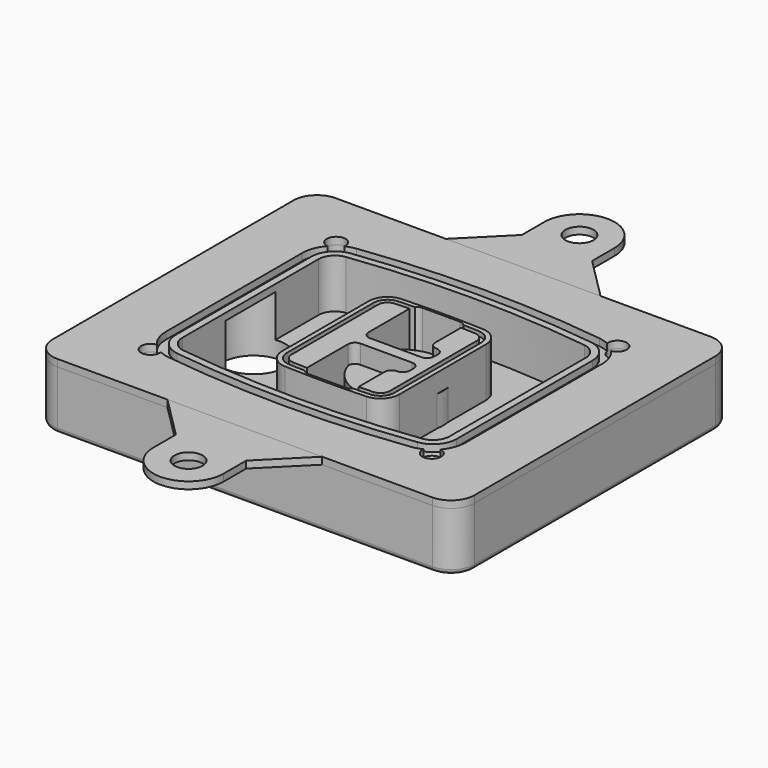
from build123d import *

# Parameters (mm, degrees)
F1_DEPTH  = 25
F2_DEPTH  = 3
F3_DEPTH  = 18
F5_DEPTH  = 21
F6_DEPTH  = 2
F8_DEPTH  = 20
F9_DEPTH  = 16
F10_DEPTH = 25
F7_R      = 6
F7_R_2    = 4
F11_DEPTH = 6
F13_DEPTH = 9
F15_R     = 2
F17_DEPTH = 3
F16_R     = 6


# Not quite as in the source:
# - a feature of the source that left no trace in its solid (it failed there, or was rolled back) is left out
# - a feature names something its author has since deleted; it is built from what else it names


with BuildPart() as f1:
    # F0 (on Top) → F1 (new body)
    with BuildSketch(Plane.XY):
        with BuildLine():
            ThreePointArc((-90, -64.25), (-87.0710678119, -71.3210678119), (-80, -74.25))
            Line((-80, -74.25), (80, -74.25))
            ThreePointArc((80, -74.25), (87.0710678119, -71.3210678119), (90, -64.25))
            Line((90, -64.25), (90, 64.25))
            ThreePointArc((90, 64.25), (87.0710678119, 71.3210678119), (80, 74.25))
            Line((80, 74.25), (-80, 74.25))
            ThreePointArc((-80, 74.25), (-87.0710678119, 71.3210678119), (-90, 64.25))
            Line((-90, 64.25), (-90, -64.25))
        make_face()
        with BuildLine():
            ThreePointArc((-60.5228833457, 45.5343231338), (-62.6370880358, 52.5076181093), (-56, 49.5))
            ThreePointArc((-56, 49.5), (-56.010223193, 49.2142010667), (-56.0408405151, 48.9298630223))
            ThreePointArc((-56.0408405151, 48.9298630223), (-53.9627965672, 49.7276492937), (-51.7845761632, 50.1860000938))
            ThreePointArc((-51.7845761632, 50.1860000938), (0, 53.5), (51.7845761632, 50.1860000938))
            ThreePointArc((51.7845761632, 50.1860000938), (53.9627965672, 49.7276492937), (56.0408405151, 48.9298630223))
            ThreePointArc((56.0408405151, 48.9298630223), (59.7142010667, 53.489776807), (64, 49.5))
            ThreePointArc((64, 49.5), (63.0076181093, 46.8629119642), (60.5228833457, 45.5343231338))
            ThreePointArc((60.5228833457, 45.5343231338), (63.1019152577, 41.2337455934), (64, 36.300205629))
            Line((64, 36.300205629), (64, -36.300205629))
            ThreePointArc((64, -36.300205629), (63.1019152577, -41.2337455934), (60.5228833457, -45.5343231338))
            ThreePointArc((60.5228833457, -45.5343231338), (63.0076181093, -46.8629119642), (64, -49.5))
            ThreePointArc((64, -49.5), (59.7142010667, -53.489776807), (56.0408405151, -48.9298630223))
            ThreePointArc((56.0408405151, -48.9298630223), (53.9627965672, -49.7276492937), (51.7845761632, -50.1860000938))
            ThreePointArc((51.7845761632, -50.1860000938), (0, -53.5), (-51.7845761632, -50.1860000938))
            ThreePointArc((-51.7845761632, -50.1860000938), (-53.9627965672, -49.7276492937), (-56.0408405151, -48.9298630223))
            ThreePointArc((-56.0408405151, -48.9298630223), (-56.010223193, -49.2142010667), (-56, -49.5))
            ThreePointArc((-56, -49.5), (-62.6370880358, -52.5076181093), (-60.5228833457, -45.5343231338))
            ThreePointArc((-60.5228833457, -45.5343231338), (-63.1019152577, -41.2337455934), (-64, -36.300205629))
            Line((-64, -36.300205629), (-64, 36.300205629))
            ThreePointArc((-64, 36.300205629), (-63.1019152577, 41.2337455934), (-60.5228833457, 45.5343231338))
        make_face(mode=Mode.SUBTRACT)
        with BuildLine():
            ThreePointArc((-56.0408405151, 48.9298630223), (-57.584545341, 46.3116495189), (-60.5228833457, 45.5343231338))
            ThreePointArc((-60.5228833457, 45.5343231338), (-63.1019152577, 41.2337455934), (-64, 36.300205629))
            Line((-64, 36.300205629), (-64, -36.300205629))
            ThreePointArc((-64, -36.300205629), (-63.1019152577, -41.2337455934), (-60.5228833457, -45.5343231338))
            ThreePointArc((-60.5228833457, -45.5343231338), (-57.584545341, -46.3116495189), (-56.0408405151, -48.9298630223))
            ThreePointArc((-56.0408405151, -48.9298630223), (-53.9627965672, -49.7276492937), (-51.7845761632, -50.1860000938))
            ThreePointArc((-51.7845761632, -50.1860000938), (0, -53.5), (51.7845761632, -50.1860000938))
            ThreePointArc((51.7845761632, -50.1860000938), (53.9627965672, -49.7276492937), (56.0408405151, -48.9298630223))
            ThreePointArc((56.0408405151, -48.9298630223), (57.584545341, -46.3116495189), (60.5228833457, -45.5343231338))
            ThreePointArc((60.5228833457, -45.5343231338), (63.1019152577, -41.2337455934), (64, -36.300205629))
            Line((64, -36.300205629), (64, 36.300205629))
            ThreePointArc((64, 36.300205629), (63.1019152577, 41.2337455934), (60.5228833457, 45.5343231338))
            ThreePointArc((60.5228833457, 45.5343231338), (57.584545341, 46.3116495189), (56.0408405151, 48.9298630223))
            ThreePointArc((56.0408405151, 48.9298630223), (53.9627965672, 49.7276492937), (51.7845761632, 50.1860000938))
            ThreePointArc((51.7845761632, 50.1860000938), (0, 53.5), (-51.7845761632, 50.1860000938))
            ThreePointArc((-51.7845761632, 50.1860000938), (-53.9627965672, 49.7276492937), (-56.0408405151, 48.9298630223))
        make_face()
        with BuildLine():
            Line((-60, -36.300205629), (-60, 36.300205629))
            ThreePointArc((-60, 36.300205629), (-57.5082279066, 42.9052426239), (-51.2746972594, 46.2186302467))
            ThreePointArc((-51.2746972594, 46.2186302467), (0, 49.5), (51.2746972594, 46.2186302467))
            ThreePointArc((51.2746972594, 46.2186302467), (57.5082279066, 42.9052426239), (60, 36.300205629))
            Line((60, 36.300205629), (60, -36.300205629))
            ThreePointArc((60, -36.300205629), (57.5082279066, -42.9052426239), (51.2746972594, -46.2186302467))
            ThreePointArc((51.2746972594, -46.2186302467), (0, -49.5), (-51.2746972594, -46.2186302467))
            ThreePointArc((-51.2746972594, -46.2186302467), (-57.5082279066, -42.9052426239), (-60, -36.300205629))
        make_face(mode=Mode.SUBTRACT)
        with BuildLine():
            ThreePointArc((-51.2746972594, 46.2186302467), (-57.5082279066, 42.9052426239), (-60, 36.300205629))
            Line((-60, 36.300205629), (-60, -36.300205629))
            ThreePointArc((-60, -36.300205629), (-57.5082279066, -42.9052426239), (-51.2746972594, -46.2186302467))
            ThreePointArc((-51.2746972594, -46.2186302467), (0, -49.5), (51.2746972594, -46.2186302467))
            ThreePointArc((51.2746972594, -46.2186302467), (57.5082279066, -42.9052426239), (60, -36.300205629))
            Line((60, -36.300205629), (60, 36.300205629))
            ThreePointArc((60, 36.300205629), (57.5082279066, 42.9052426239), (51.2746972594, 46.2186302467))
            ThreePointArc((51.2746972594, 46.2186302467), (0, 49.5), (-51.2746972594, 46.2186302467))
        make_face()
        with BuildLine():
            ThreePointArc((50.8922880816, 43.2431028614), (55.2557595346, 40.9237315254), (57, 36.300205629))
            Line((57, 36.300205629), (57, -36.300205629))
            ThreePointArc((57, -36.300205629), (55.2557595346, -40.9237315254), (50.8922880816, -43.2431028614))
            ThreePointArc((50.8922880816, -43.2431028614), (0, -46.5), (-50.8922880816, -43.2431028614))
            ThreePointArc((-50.8922880816, -43.2431028614), (-55.2557595346, -40.9237315254), (-57, -36.300205629))
            Line((-57, -36.300205629), (-57, 36.300205629))
            ThreePointArc((-57, 36.300205629), (-55.2557595346, 40.9237315254), (-50.8922880816, 43.2431028614))
            ThreePointArc((-50.8922880816, 43.2431028614), (0, 46.5), (50.8922880816, 43.2431028614))
        make_face(mode=Mode.SUBTRACT)
        with BuildLine():
            Line((57, -36.300205629), (57, 36.300205629))
            ThreePointArc((57, 36.300205629), (55.2557595346, 40.9237315254), (50.8922880816, 43.2431028614))
            ThreePointArc((50.8922880816, 43.2431028614), (0, 46.5), (-50.8922880816, 43.2431028614))
            ThreePointArc((-50.8922880816, 43.2431028614), (-55.2557595346, 40.9237315254), (-57, 36.300205629))
            Line((-57, 36.300205629), (-57, -36.300205629))
            ThreePointArc((-57, -36.300205629), (-55.2557595346, -40.9237315254), (-50.8922880816, -43.2431028614))
            ThreePointArc((-50.8922880816, -43.2431028614), (0, -46.5), (50.8922880816, -43.2431028614))
            ThreePointArc((50.8922880816, -43.2431028614), (55.2557595346, -40.9237315254), (57, -36.300205629))
        make_face()
    extrude(amount=-F1_DEPTH)

    # F0 (on Top) → F2 (join)
    with BuildSketch(Plane.XY):
        with BuildLine():
            ThreePointArc((-51.2746972594, 46.2186302467), (-57.5082279066, 42.9052426239), (-60, 36.300205629))
            Line((-60, 36.300205629), (-60, -36.300205629))
            ThreePointArc((-60, -36.300205629), (-57.5082279066, -42.9052426239), (-51.2746972594, -46.2186302467))
            ThreePointArc((-51.2746972594, -46.2186302467), (0, -49.5), (51.2746972594, -46.2186302467))
            ThreePointArc((51.2746972594, -46.2186302467), (57.5082279066, -42.9052426239), (60, -36.300205629))
            Line((60, -36.300205629), (60, 36.300205629))
            ThreePointArc((60, 36.300205629), (57.5082279066, 42.9052426239), (51.2746972594, 46.2186302467))
            ThreePointArc((51.2746972594, 46.2186302467), (0, 49.5), (-51.2746972594, 46.2186302467))
        make_face()
        with BuildLine():
            ThreePointArc((50.8922880816, 43.2431028614), (55.2557595346, 40.9237315254), (57, 36.300205629))
            Line((57, 36.300205629), (57, -36.300205629))
            ThreePointArc((57, -36.300205629), (55.2557595346, -40.9237315254), (50.8922880816, -43.2431028614))
            ThreePointArc((50.8922880816, -43.2431028614), (0, -46.5), (-50.8922880816, -43.2431028614))
            ThreePointArc((-50.8922880816, -43.2431028614), (-55.2557595346, -40.9237315254), (-57, -36.300205629))
            Line((-57, -36.300205629), (-57, 36.300205629))
            ThreePointArc((-57, 36.300205629), (-55.2557595346, 40.9237315254), (-50.8922880816, 43.2431028614))
            ThreePointArc((-50.8922880816, 43.2431028614), (0, 46.5), (50.8922880816, 43.2431028614))
        make_face(mode=Mode.SUBTRACT)
    extrude(amount=F2_DEPTH)

    # F0 (on Top) → F3 (cut)
    with BuildSketch(Plane.XY):
        with BuildLine():
            Line((57, -36.300205629), (57, 36.300205629))
            ThreePointArc((57, 36.300205629), (55.2557595346, 40.9237315254), (50.8922880816, 43.2431028614))
            ThreePointArc((50.8922880816, 43.2431028614), (0, 46.5), (-50.8922880816, 43.2431028614))
            ThreePointArc((-50.8922880816, 43.2431028614), (-55.2557595346, 40.9237315254), (-57, 36.300205629))
            Line((-57, 36.300205629), (-57, -36.300205629))
            ThreePointArc((-57, -36.300205629), (-55.2557595346, -40.9237315254), (-50.8922880816, -43.2431028614))
            ThreePointArc((-50.8922880816, -43.2431028614), (0, -46.5), (50.8922880816, -43.2431028614))
            ThreePointArc((50.8922880816, -43.2431028614), (55.2557595346, -40.9237315254), (57, -36.300205629))
        make_face()
    extrude(amount=-F3_DEPTH, mode=Mode.SUBTRACT)

    # F4 (on face) → F5 (join, through all)
    with BuildSketch(Plane.XY.offset(3)):
        with BuildLine():
            ThreePointArc((-25, -23.1157506345), (-22.7832384679, -28.6433317351), (-17.361461794, -31.1075805483))
            ThreePointArc((-17.361461794, -31.1075805483), (0, -31.5), (17.361461794, -31.1075805483))
            ThreePointArc((17.361461794, -31.1075805483), (22.7832384679, -28.6433317351), (25, -23.1157506345))
            Line((25, -23.1157506345), (25, 23.1157506345))
            ThreePointArc((25, 23.1157506345), (22.7832384679, 28.6433317351), (17.361461794, 31.1075805483))
            ThreePointArc((17.361461794, 31.1075805483), (0, 31.5), (-17.361461794, 31.1075805483))
            ThreePointArc((-17.361461794, 31.1075805483), (-22.7832384679, 28.6433317351), (-25, 23.1157506345))
            Line((-25, 23.1157506345), (-25, -23.1157506345))
        make_face()
        with BuildLine():
            ThreePointArc((17.2710963455, 29.1096230698), (21.3374288509, 27.2614364599), (23, 23.1157506345))
            Line((23, 23.1157506345), (23, -23.1157506345))
            ThreePointArc((23, -23.1157506345), (21.3374288509, -27.2614364599), (17.2710963455, -29.1096230698))
            ThreePointArc((17.2710963455, -29.1096230698), (13.8131178726, -29.2503406735), (10.354007104, -29.3597447552))
            ThreePointArc((10.354007104, -29.3597447552), (9.3078160678, -30.1999290977), (8, -30.5))
            Line((8, -30.5), (-8, -30.5))
            ThreePointArc((-8, -30.5), (-9.3078160678, -30.1999290977), (-10.354007104, -29.3597447552))
            ThreePointArc((-10.354007104, -29.3597447552), (-13.8131178726, -29.2503406735), (-17.2710963455, -29.1096230698))
            ThreePointArc((-17.2710963455, -29.1096230698), (-21.3374288509, -27.2614364599), (-23, -23.1157506345))
            Line((-23, -23.1157506345), (-23, 23.1157506345))
            ThreePointArc((-23, 23.1157506345), (-21.3374288509, 27.2614364599), (-17.2710963455, 29.1096230698))
            ThreePointArc((-17.2710963455, 29.1096230698), (-13.8131178726, 29.2503406735), (-10.354007104, 29.3597447552))
            ThreePointArc((-10.354007104, 29.3597447552), (-9.3078160678, 30.1999290977), (-8, 30.5))
            Line((-8, 30.5), (8, 30.5))
            ThreePointArc((8, 30.5), (9.3078160678, 30.1999290977), (10.354007104, 29.3597447552))
            ThreePointArc((10.354007104, 29.3597447552), (13.8131178726, 29.2503406735), (17.2710963455, 29.1096230698))
        make_face(mode=Mode.SUBTRACT)
        with BuildLine():
            Line((23, -23.1157506345), (23, 23.1157506345))
            ThreePointArc((23, 23.1157506345), (21.3374288509, 27.2614364599), (17.2710963455, 29.1096230698))
            ThreePointArc((17.2710963455, 29.1096230698), (13.8131178726, 29.2503406735), (10.354007104, 29.3597447552))
            ThreePointArc((10.354007104, 29.3597447552), (10.8339037838, 28.4843725637), (11, 27.5))
            Line((11, 27.5), (11, 27.3408608478))
            ThreePointArc((11, 27.3408608478), (14.0908314548, 27.2388300581), (17.180730897, 27.1116655914))
            ThreePointArc((17.180730897, 27.1116655914), (19.8916192339, 25.8795411848), (21, 23.1157506345))
            Line((21, 23.1157506345), (21, -23.1157506345))
            ThreePointArc((21, -23.1157506345), (19.8916192339, -25.8795411848), (17.180730897, -27.1116655914))
            ThreePointArc((17.180730897, -27.1116655914), (14.0908314548, -27.2388300581), (11, -27.3408608478))
            Line((11, -27.3408608478), (11, -27.5))
            ThreePointArc((11, -27.5), (10.8339037838, -28.4843725637), (10.354007104, -29.3597447552))
            ThreePointArc((10.354007104, -29.3597447552), (13.8131178726, -29.2503406735), (17.2710963455, -29.1096230698))
            ThreePointArc((17.2710963455, -29.1096230698), (21.3374288509, -27.2614364599), (23, -23.1157506345))
        make_face()
        with BuildLine():
            ThreePointArc((17.180730897, 27.1116655914), (14.0908314548, 27.2388300581), (11, 27.3408608478))
            Line((11, 27.3408608478), (11, 13.5))
            ThreePointArc((11, 13.5), (11.8786796564, 11.3786796564), (14, 10.5))
            ThreePointArc((14, 10.5), (16.1213203436, 9.6213203436), (17, 7.5))
            Line((17, 7.5), (17, 5.5))
            ThreePointArc((17, 5.5), (16.1213203436, 3.3786796564), (14, 2.5))
            Line((14, 2.5), (-8, 2.5))
            ThreePointArc((-8, 2.5), (-10.1213203436, 3.3786796564), (-11, 5.5))
            Line((-11, 5.5), (-11, 27.3408608478))
            ThreePointArc((-11, 27.3408608478), (-14.0908314548, 27.2388300581), (-17.180730897, 27.1116655914))
            ThreePointArc((-17.180730897, 27.1116655914), (-19.8916192339, 25.8795411848), (-21, 23.1157506345))
            Line((-21, 23.1157506345), (-21, -23.1157506345))
            ThreePointArc((-21, -23.1157506345), (-19.8916192339, -25.8795411848), (-17.180730897, -27.1116655914))
            ThreePointArc((-17.180730897, -27.1116655914), (-14.0908314548, -27.2388300581), (-11, -27.3408608478))
            Line((-11, -27.3408608478), (-11, -5.5))
            ThreePointArc((-11, -5.5), (-10.1213203436, -3.3786796564), (-8, -2.5))
            Line((-8, -2.5), (14, -2.5))
            ThreePointArc((14, -2.5), (16.1213203436, -3.3786796564), (17, -5.5))
            Line((17, -5.5), (17, -7.5))
            ThreePointArc((17, -7.5), (16.1213203436, -9.6213203436), (14, -10.5))
            ThreePointArc((14, -10.5), (11.8786796564, -11.3786796564), (11, -13.5))
            Line((11, -13.5), (11, -27.3408608478))
            ThreePointArc((11, -27.3408608478), (14.0908314548, -27.2388300581), (17.180730897, -27.1116655914))
            ThreePointArc((17.180730897, -27.1116655914), (19.8916192339, -25.8795411848), (21, -23.1157506345))
            Line((21, -23.1157506345), (21, 23.1157506345))
            ThreePointArc((21, 23.1157506345), (19.8916192339, 25.8795411848), (17.180730897, 27.1116655914))
        make_face()
    extrude(amount=-F5_DEPTH)

    # F4 (on face) → F6 (cut)
    with BuildSketch(Plane.XY.offset(3)):
        with BuildLine():
            Line((23, -23.1157506345), (23, 23.1157506345))
            ThreePointArc((23, 23.1157506345), (21.3374288509, 27.2614364599), (17.2710963455, 29.1096230698))
            ThreePointArc((17.2710963455, 29.1096230698), (13.8131178726, 29.2503406735), (10.354007104, 29.3597447552))
            ThreePointArc((10.354007104, 29.3597447552), (10.8339037838, 28.4843725637), (11, 27.5))
            Line((11, 27.5), (11, 27.3408608478))
            ThreePointArc((11, 27.3408608478), (14.0908314548, 27.2388300581), (17.180730897, 27.1116655914))
            ThreePointArc((17.180730897, 27.1116655914), (19.8916192339, 25.8795411848), (21, 23.1157506345))
            Line((21, 23.1157506345), (21, -23.1157506345))
            ThreePointArc((21, -23.1157506345), (19.8916192339, -25.8795411848), (17.180730897, -27.1116655914))
            ThreePointArc((17.180730897, -27.1116655914), (14.0908314548, -27.2388300581), (11, -27.3408608478))
            Line((11, -27.3408608478), (11, -27.5))
            ThreePointArc((11, -27.5), (10.8339037838, -28.4843725637), (10.354007104, -29.3597447552))
            ThreePointArc((10.354007104, -29.3597447552), (13.8131178726, -29.2503406735), (17.2710963455, -29.1096230698))
            ThreePointArc((17.2710963455, -29.1096230698), (21.3374288509, -27.2614364599), (23, -23.1157506345))
        make_face()
    extrude(amount=-F6_DEPTH, mode=Mode.SUBTRACT)

    # F7 (on face) → F8 (join)
    with BuildSketch(Plane(origin=(0, 0, -25), x_dir=(1, 0, 0), z_dir=(0, 0, -1))):
        with BuildLine():
            ThreePointArc((-6.71157564, 0), (6.7567035675, 13.4682792075), (20.224982775, 0))
            Line((20.224982775, 0), (25.224982775, 0))
            ThreePointArc((25.224982775, 0), (6.7567035675, 18.4682792075), (-11.71157564, 0))
            Line((-11.71157564, 0), (-6.71157564, 0))
        make_face()
        with BuildLine():
            Line((-6.71157564, 0), (20.224982775, 0))
            ThreePointArc((20.224982775, 0), (6.7567035675, 13.4682792075), (-6.71157564, 0))
        make_face()
        with BuildLine():
            ThreePointArc((-6.71157564, 0), (6.7567035675, -13.4682792075), (20.224982775, 0))
            Line((20.224982775, 0), (-6.71157564, 0))
        make_face()
        with BuildLine():
            Line((25.224982775, 0), (20.224982775, 0))
            ThreePointArc((20.224982775, 0), (6.7567035675, -13.4682792075), (-6.71157564, 0))
            Line((-6.71157564, 0), (-11.71157564, 0))
            ThreePointArc((-11.71157564, 0), (6.7567035675, -18.4682792075), (25.224982775, 0))
        make_face()
    extrude(amount=-F8_DEPTH)

    # F7 (on face) → F9 (cut)
    with BuildSketch(Plane(origin=(0, 0, -25), x_dir=(1, 0, 0), z_dir=(0, 0, -1))):
        with BuildLine():
            Line((-6.71157564, 0), (20.224982775, 0))
            ThreePointArc((20.224982775, 0), (6.7567035675, 13.4682792075), (-6.71157564, 0))
        make_face()
        with BuildLine():
            ThreePointArc((-6.71157564, 0), (6.7567035675, -13.4682792075), (20.224982775, 0))
            Line((20.224982775, 0), (-6.71157564, 0))
        make_face()
    extrude(amount=-F9_DEPTH, mode=Mode.SUBTRACT)

    # F7 (on face) → F10 (cut)
    with BuildSketch(Plane(origin=(0, 0, -25), x_dir=(1, 0, 0), z_dir=(0, 0, -1))):
        with BuildLine():
            Line((-69.0318229325, 0), (-42.0952645175, 0))
            ThreePointArc((-42.0952645175, 0), (-55.563543725, 13.4682792075), (-69.0318229325, 0))
        make_face()
        with BuildLine():
            ThreePointArc((-69.0318229325, 0), (-55.563543725, -13.4682792075), (-42.0952645175, 0))
            Line((-42.0952645175, 0), (-69.0318229325, 0))
        make_face()
    extrude(amount=-F10_DEPTH, mode=Mode.SUBTRACT)

    # F7 (on face) → F11 (cut)
    with BuildSketch(Plane(origin=(0, 0, -25), x_dir=(1, 0, 0), z_dir=(0, 0, -1))):
        with Locations((60, -49.5)):
            Circle(F7_R)
        with Locations((60, -49.5)):
            Circle(F7_R_2, mode=Mode.SUBTRACT)
        with Locations((-60, -49.5)):
            Circle(F7_R)
        with Locations((-60, -49.5)):
            Circle(F7_R_2, mode=Mode.SUBTRACT)
        with Locations((-60, 49.5)):
            Circle(F7_R)
        with Locations((-60, 49.5)):
            Circle(F7_R_2, mode=Mode.SUBTRACT)
        with Locations((60, 49.5)):
            Circle(F7_R)
        with Locations((60, 49.5)):
            Circle(F7_R_2, mode=Mode.SUBTRACT)
    extrude(amount=-F11_DEPTH, mode=Mode.SUBTRACT)

    # F12 (on face) → F13 (cut, through all)
    with BuildSketch(Plane(origin=(0, 0, -9), x_dir=(1, 0, 0), z_dir=(0, 0, -1))):
        with BuildLine():
            ThreePointArc((20.224982775, 0), (20.1663399806, 1.2554664788), (19.9909222755, 2.5))
            Line((19.9909222755, 2.5), (14, 2.5))
            ThreePointArc((14, 2.5), (16.1213203436, 3.3786796564), (17, 5.5))
            Line((17, 5.5), (17, 7.5))
            ThreePointArc((17, 7.5), (16.1213203436, 9.6213203436), (14, 10.5))
            ThreePointArc((14, 10.5), (12.1627255951, 11.1284134507), (11.0951631559, 12.750384826))
            ThreePointArc((11.0951631559, 12.750384826), (11.0476113807, 12.7664660322), (11, 12.7823698976))
            Line((11, 12.7823698976), (11, -12.7823698976))
            ThreePointArc((11, -12.7823698976), (11.0476113807, -12.7664660322), (11.0951631559, -12.750384826))
            ThreePointArc((11.0951631559, -12.750384826), (12.1627255951, -11.1284134507), (14, -10.5))
            ThreePointArc((14, -10.5), (16.1213203436, -9.6213203436), (17, -7.5))
            Line((17, -7.5), (17, -5.5))
            ThreePointArc((17, -5.5), (16.1213203436, -3.3786796564), (14, -2.5))
            Line((14, -2.5), (19.9909222755, -2.5))
            ThreePointArc((19.9909222755, -2.5), (20.1663399806, -1.2554664788), (20.224982775, 0))
        make_face()
    extrude(amount=F13_DEPTH, mode=Mode.SUBTRACT)

    # F15
    f15_edges = [f1.edges().sort_by_distance(p)[0] for p in [
        (0, -74.25, -25),
        (-87.071068, -71.321068, -25),
        (-90, 0, -25),
        (-87.071068, 71.321068, -25),
        (87.071068, -71.321068, -25),
        (0, 74.25, -25),
        (90, 0, -25),
        (87.071068, 71.321068, -25),
    ]]
    fillet(f15_edges, radius=F15_R)


with BuildPart() as f17:
    # F0 (on Top) → F17 (new body, through all)
    with BuildSketch(Plane.XY):
        with BuildLine():
            ThreePointArc((-90, -64.25), (-87.0710678119, -71.3210678119), (-80, -74.25))
            Line((-80, -74.25), (80, -74.25))
            ThreePointArc((80, -74.25), (87.0710678119, -71.3210678119), (90, -64.25))
            Line((90, -64.25), (90, 64.25))
            ThreePointArc((90, 64.25), (87.0710678119, 71.3210678119), (80, 74.25))
            Line((80, 74.25), (-80, 74.25))
            ThreePointArc((-80, 74.25), (-87.0710678119, 71.3210678119), (-90, 64.25))
            Line((-90, 64.25), (-90, -64.25))
        make_face()
        with BuildLine():
            ThreePointArc((-60.5228833457, 45.5343231338), (-62.6370880358, 52.5076181093), (-56, 49.5))
            ThreePointArc((-56, 49.5), (-56.010223193, 49.2142010667), (-56.0408405151, 48.9298630223))
            ThreePointArc((-56.0408405151, 48.9298630223), (-53.9627965672, 49.7276492937), (-51.7845761632, 50.1860000938))
            ThreePointArc((-51.7845761632, 50.1860000938), (0, 53.5), (51.7845761632, 50.1860000938))
            ThreePointArc((51.7845761632, 50.1860000938), (53.9627965672, 49.7276492937), (56.0408405151, 48.9298630223))
            ThreePointArc((56.0408405151, 48.9298630223), (59.7142010667, 53.489776807), (64, 49.5))
            ThreePointArc((64, 49.5), (63.0076181093, 46.8629119642), (60.5228833457, 45.5343231338))
            ThreePointArc((60.5228833457, 45.5343231338), (63.1019152577, 41.2337455934), (64, 36.300205629))
            Line((64, 36.300205629), (64, -36.300205629))
            ThreePointArc((64, -36.300205629), (63.1019152577, -41.2337455934), (60.5228833457, -45.5343231338))
            ThreePointArc((60.5228833457, -45.5343231338), (63.0076181093, -46.8629119642), (64, -49.5))
            ThreePointArc((64, -49.5), (59.7142010667, -53.489776807), (56.0408405151, -48.9298630223))
            ThreePointArc((56.0408405151, -48.9298630223), (53.9627965672, -49.7276492937), (51.7845761632, -50.1860000938))
            ThreePointArc((51.7845761632, -50.1860000938), (0, -53.5), (-51.7845761632, -50.1860000938))
            ThreePointArc((-51.7845761632, -50.1860000938), (-53.9627965672, -49.7276492937), (-56.0408405151, -48.9298630223))
            ThreePointArc((-56.0408405151, -48.9298630223), (-56.010223193, -49.2142010667), (-56, -49.5))
            ThreePointArc((-56, -49.5), (-62.6370880358, -52.5076181093), (-60.5228833457, -45.5343231338))
            ThreePointArc((-60.5228833457, -45.5343231338), (-63.1019152577, -41.2337455934), (-64, -36.300205629))
            Line((-64, -36.300205629), (-64, 36.300205629))
            ThreePointArc((-64, 36.300205629), (-63.1019152577, 41.2337455934), (-60.5228833457, 45.5343231338))
        make_face(mode=Mode.SUBTRACT)
    extrude(amount=F17_DEPTH)


with BuildPart() as f17b:
    # F16 (on face) → F17, piece 2 (new body, through all)
    with BuildSketch(Plane.XY):
        with BuildLine():
            ThreePointArc((15, 104.25), (0, 119.25), (-15, 104.25))
            Line((-15, 104.25), (-15, 92.25))
            Line((-15, 92.25), (-33, 74.25))
            Line((-33, 74.25), (33, 74.25))
            Line((33, 74.25), (15, 92.25))
            Line((15, 92.25), (15, 104.25))
        make_face()
        with Locations((0, 104.25)):
            Circle(F16_R, mode=Mode.SUBTRACT)
    extrude(amount=F17_DEPTH)


with BuildPart() as f17c:
    # F16 (on face) → F17, piece 3 (new body, through all)
    with BuildSketch(Plane.XY):
        with BuildLine():
            Line((33, -74.25), (-33, -74.25))
            Line((-33, -74.25), (-15, -92.25))
            Line((-15, -92.25), (-15, -104.25))
            ThreePointArc((-15, -104.25), (0, -119.25), (15, -104.25))
            Line((15, -104.25), (15, -92.25))
            Line((15, -92.25), (33, -74.25))
        make_face()
        with Locations((0, -104.25)):
            Circle(F16_R, mode=Mode.SUBTRACT)
    extrude(amount=F17_DEPTH)


solid = Compound([f1.part, f17.part, f17b.part, f17c.part])
